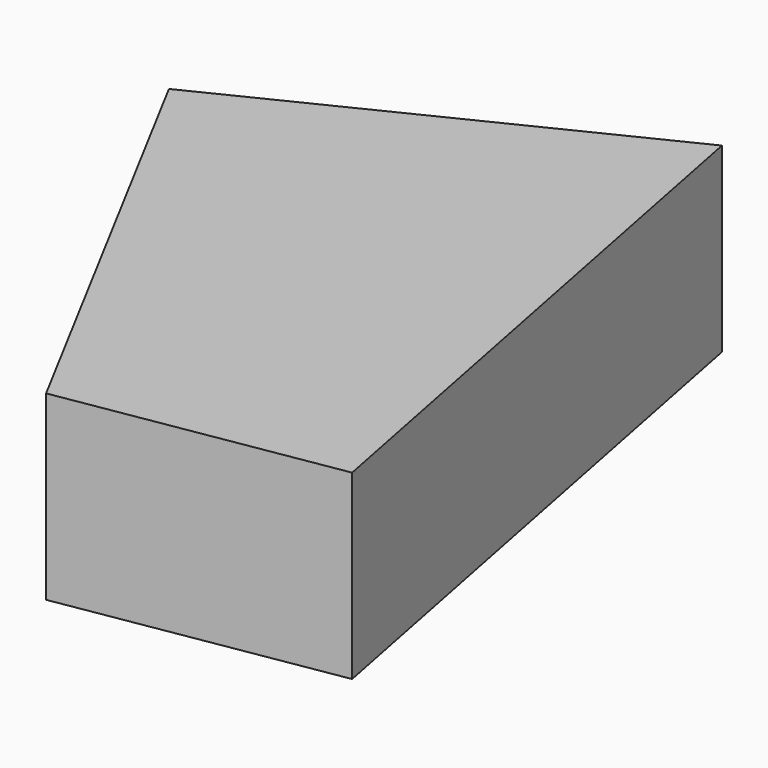
from build123d import *

# Parameters (mm, degrees)
F3_DEPTH = 25.4


# Not quite as in the source:
# - the program builds the solid bodies; features that only make, move or delete a surface that nothing else refers to are left out


with BuildPart() as f3:
    # F2 (on Top) → F3 (new body)
    with BuildSketch(Plane.XY):
        Polygon((16.5086686611, -58.330655098), (-0.272778012, 27.2547331593), (-55.7626336813, 0), (-21.2778449059, -64.5672678947), align=None)
    extrude(amount=F3_DEPTH)


solid = f3.part
